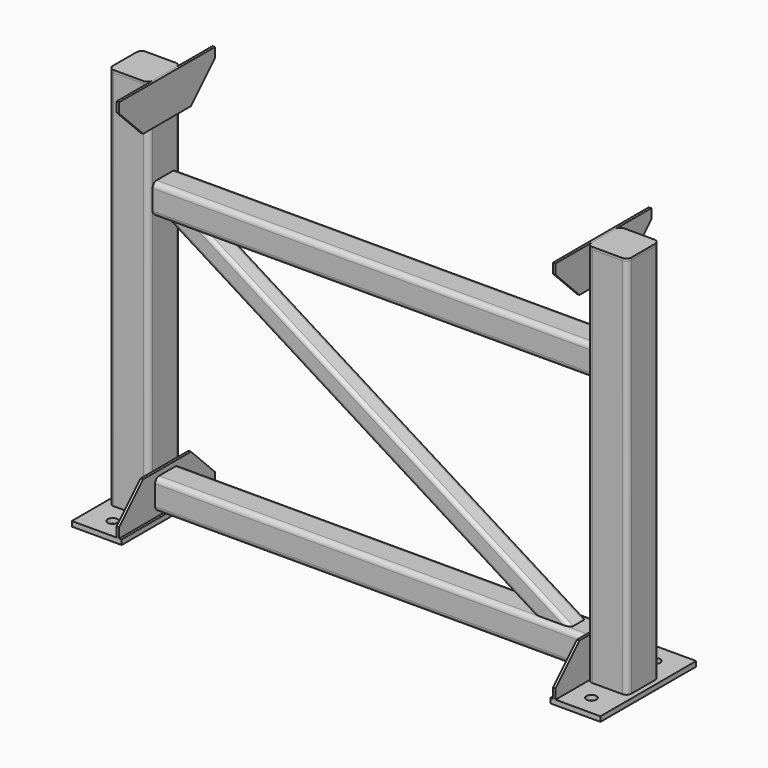
from build123d import *

# Parameters (mm, degrees)
F0_W      = 127
F0_H      = 304.8
F0_R      = 12.7
F1_DEPTH  = 12.7
F3_DEPTH  = 971.55
F5_DEPTH  = 6.35
F7_DEPTH  = 6.35
F12_DEPTH = 1117.6
F15_DEPTH = 25.4
F16_R     = 9.652


with BuildPart() as f1:
    # F0 (on Top) → F1 (new body)
    with BuildSketch(Plane.XY):
        with Locations((-609.6, 0)):
            Rectangle(F0_W, F0_H)
        with Locations((-609.6, -101.6)):
            Circle(F0_R, mode=Mode.SUBTRACT)
        with Locations((-609.6, 101.6)):
            Circle(F0_R, mode=Mode.SUBTRACT)
    extrude(amount=F1_DEPTH)

    # F2 (on face) → F3 (join)
    with BuildSketch(Plane.XY.offset(12.7)):
        with BuildLine():
            Line((-571.5, 50.8), (-647.7, 50.8))
            ThreePointArc((-647.7, 50.8), (-656.6802561211, 47.0802561211), (-660.4, 38.1))
            Line((-660.4, 38.1), (-660.4, -38.1))
            ThreePointArc((-660.4, -38.1), (-656.6802561211, -47.0802561211), (-647.7, -50.8))
            Line((-647.7, -50.8), (-571.5, -50.8))
            ThreePointArc((-571.5, -50.8), (-562.5197438789, -47.0802561211), (-558.8, -38.1))
            Line((-558.8, -38.1), (-558.8, 38.1))
            ThreePointArc((-558.8, 38.1), (-562.5197438789, 47.0802561211), (-571.5, 50.8))
        make_face()
        with BuildLine():
            ThreePointArc((-654.05, 38.1), (-652.1901280605, 42.5901280605), (-647.7, 44.45))
            Line((-647.7, 44.45), (-571.5, 44.45))
            ThreePointArc((-571.5, 44.45), (-567.0098719395, 42.5901280605), (-565.15, 38.1))
            Line((-565.15, 38.1), (-565.15, -38.1))
            ThreePointArc((-565.15, -38.1), (-567.0098719395, -42.5901280605), (-571.5, -44.45))
            Line((-571.5, -44.45), (-647.7, -44.45))
            ThreePointArc((-647.7, -44.45), (-652.1901280605, -42.5901280605), (-654.05, -38.1))
            Line((-654.05, -38.1), (-654.05, 38.1))
        make_face(mode=Mode.SUBTRACT)
    extrude(amount=F3_DEPTH)


with BuildPart() as f5:
    # F4 (on face) → F5 (new body)
    with BuildSketch(Plane.XY.offset(984.25)):
        with BuildLine():
            ThreePointArc((-647.7, 50.8), (-656.6802561211, 47.0802561211), (-660.4, 38.1))
            Line((-660.4, 38.1), (-660.4, -38.1))
            ThreePointArc((-660.4, -38.1), (-656.6802561211, -47.0802561211), (-647.7, -50.8))
            Line((-647.7, -50.8), (-571.5, -50.8))
            ThreePointArc((-571.5, -50.8), (-562.5197438789, -47.0802561211), (-558.8, -38.1))
            Line((-558.8, -38.1), (-558.8, 38.1))
            ThreePointArc((-558.8, 38.1), (-562.5197438789, 47.0802561211), (-571.5, 50.8))
            Line((-571.5, 50.8), (-647.7, 50.8))
        make_face()
    extrude(amount=F5_DEPTH)


with BuildPart() as f7:
    # F6 (on face) → F7 (new body)
    with BuildSketch(Plane.YZ.offset(-558.8)):
        Polygon((-152.4, 12.7), (152.4, 12.7), (152.4, 38.1), (76.2, 114.3), (-76.2, 114.3), (-152.4, 38.1), align=None)
    extrude(amount=F7_DEPTH)


with BuildPart() as f8_1:
    # F8: instance of F7
    add(f7.part.mirror(Plane(origin=(-609.6, 0, 990.6), x_dir=(1, 0, 0), z_dir=(0, 0, 1))))


with BuildPart() as f8_1_1:
    # F9: moved
    add(f8_1.part.moved(Location((0, 0, -971.55))))


with BuildPart() as f8_1_2:
    # F10: moved
    add(f8_1_1.part.moved(Location((0, 0, -6.35))))


with BuildPart() as f12:
    # F11 (on face) → F12 (new body)
    with BuildSketch(Plane.YZ.offset(-558.8)):
        with BuildLine():
            Line((25.4, 101.6), (-25.4, 101.6))
            ThreePointArc((-25.4, 101.6), (-34.3802561211, 97.8802561211), (-38.1, 88.9))
            Line((-38.1, 88.9), (-38.1, 38.1))
            ThreePointArc((-38.1, 38.1), (-34.3802561211, 29.1197438789), (-25.4, 25.4))
            Line((-25.4, 25.4), (25.4, 25.4))
            ThreePointArc((25.4, 25.4), (34.3802561211, 29.1197438789), (38.1, 38.1))
            Line((38.1, 38.1), (38.1, 88.9))
            ThreePointArc((38.1, 88.9), (34.3802561211, 97.8802561211), (25.4, 101.6))
        make_face()
        with BuildLine():
            ThreePointArc((-31.75, 88.9), (-29.8901280605, 93.3901280605), (-25.4, 95.25))
            Line((-25.4, 95.25), (25.4, 95.25))
            ThreePointArc((25.4, 95.25), (29.8901280605, 93.3901280605), (31.75, 88.9))
            Line((31.75, 88.9), (31.75, 38.1))
            ThreePointArc((31.75, 38.1), (29.8901280605, 33.6098719395), (25.4, 31.75))
            Line((25.4, 31.75), (-25.4, 31.75))
            ThreePointArc((-25.4, 31.75), (-29.8901280605, 33.6098719395), (-31.75, 38.1))
            Line((-31.75, 38.1), (-31.75, 88.9))
        make_face(mode=Mode.SUBTRACT)
    extrude(amount=F12_DEPTH)


with BuildPart() as f12b:
    # F11 (on face) → F12, piece 2 (new body)
    with BuildSketch(Plane.YZ.offset(-558.8)):
        with BuildLine():
            ThreePointArc((-25.4, 762), (-34.3802561211, 758.2802561211), (-38.1, 749.3))
            Line((-38.1, 749.3), (-38.1, 698.5))
            ThreePointArc((-38.1, 698.5), (-34.3802561211, 689.5197438789), (-25.4, 685.8))
            Line((-25.4, 685.8), (25.4, 685.8))
            ThreePointArc((25.4, 685.8), (34.3802561211, 689.5197438789), (38.1, 698.5))
            Line((38.1, 698.5), (38.1, 749.3))
            ThreePointArc((38.1, 749.3), (34.3802561211, 758.2802561211), (25.4, 762))
            Line((25.4, 762), (-25.4, 762))
        make_face()
        with BuildLine():
            ThreePointArc((25.4, 755.65), (29.8901280605, 753.7901280605), (31.75, 749.3))
            Line((31.75, 749.3), (31.75, 698.5))
            ThreePointArc((31.75, 698.5), (29.8901280605, 694.0098719395), (25.4, 692.15))
            Line((25.4, 692.15), (-25.4, 692.15))
            ThreePointArc((-25.4, 692.15), (-29.8901280605, 694.0098719395), (-31.75, 698.5))
            Line((-31.75, 698.5), (-31.75, 749.3))
            ThreePointArc((-31.75, 749.3), (-29.8901280605, 753.7901280605), (-25.4, 755.65))
            Line((-25.4, 755.65), (25.4, 755.65))
        make_face(mode=Mode.SUBTRACT)
    extrude(amount=F12_DEPTH)


with BuildPart() as f13_1:
    # F13: instance of F1
    add(f1.part.mirror(Plane.YZ))


with BuildPart() as f13_2:
    # F13: instance of F7
    add(f7.part.mirror(Plane.YZ))


with BuildPart() as f13_3:
    # F13: instance of F5
    add(f5.part.mirror(Plane.YZ))


with BuildPart() as f13_4:
    # F13: instance of F8_1
    add(f8_1_2.part.mirror(Plane.YZ))


with BuildPart() as f13_5:
    # F13: instance of F12
    add(f12.part.mirror(Plane.YZ))


with BuildPart() as f13_6:
    # F13: instance of F12b
    add(f12b.part.mirror(Plane.YZ))


with BuildPart() as f15:
    # F14 (on Front) → F15 (new body, symmetric)
    with BuildSketch(Plane.XZ):
        Polygon((494.9646241508, 101.6), (-439.7553758492, 685.8), (-535.6046241508, 685.8), (399.1153758492, 101.6), align=None)
    extrude(amount=F15_DEPTH, both=True)

    # F16
    f16_edges = [f15.edges().sort_by_distance(p)[0] for p in [
        (27.604624, -25.4, 393.7),
        (-68.244624, -25.4, 393.7),
        (27.604624, 25.4, 393.7),
        (-68.244624, 25.4, 393.7),
    ]]
    fillet(f16_edges, radius=F16_R)


solid = Compound([f1.part, f5.part, f7.part, f8_1_2.part, f12.part, f12b.part, f13_1.part, f13_2.part, f13_3.part, f13_4.part, f13_5.part, f13_6.part, f15.part])
